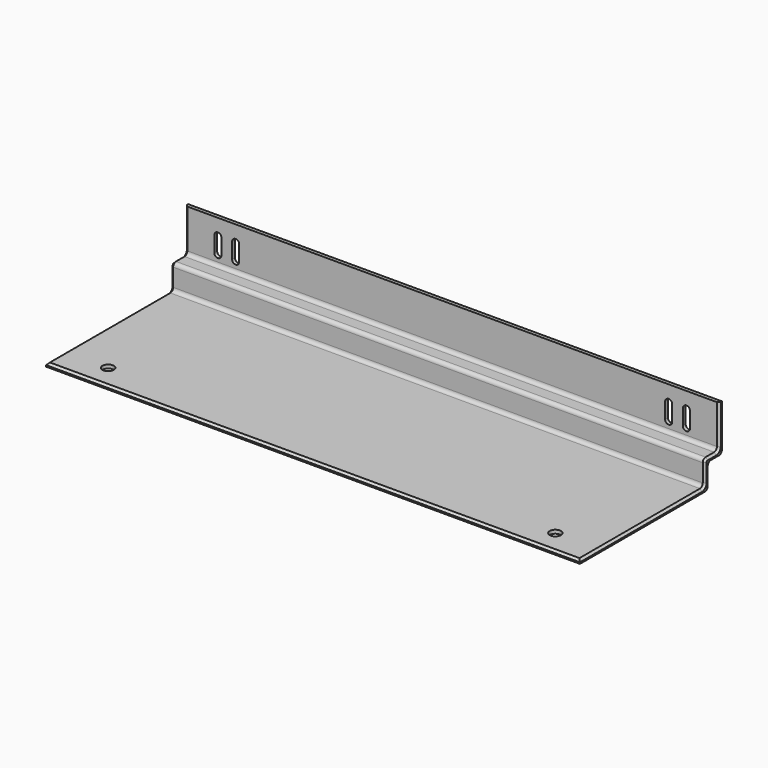
from build123d import *

# Parameters (mm, degrees)
F1_DEPTH     = 752
F3_DEPTH     = 5.001
F5_SIZE      = 3
F6_SIZE      = 3
F7_SIZE      = 3
F4_R         = 8
F8_DEPTH     = 25
F9_TEXT_SIZE = 16.7984515429
F10_DEPTH    = 0.5


# Not quite as in the source:
# - Text() gives the source's letters only with a copy of the font that has no kerning and outlines rounded to 1/6400 em; it was checked with that copy


with BuildPart() as f1:
    # F0 (on Right) → F1 (new body)
    with BuildSketch(Plane.YZ):
        with BuildLine():
            Line((0, -60), (0, 0))
            Line((0, 0), (-5, 0))
            Line((-5, 0), (-5, -55))
            ThreePointArc((-5, -55), (-6.4644660941, -58.5355339059), (-10, -60))
            Line((-10, -60), (-25, -60))
            ThreePointArc((-25, -60), (-28.5355339059, -61.4644660941), (-30, -65))
            Line((-30, -65), (-30, -90))
            ThreePointArc((-30, -90), (-31.4644660941, -93.5355339059), (-35, -95))
            Line((-35, -95), (-250, -95))
            Line((-250, -95), (-250, -100))
            Line((-250, -100), (-30, -100))
            ThreePointArc((-30, -100), (-26.4644660941, -98.5355339059), (-25, -95))
            Line((-25, -95), (-25, -70))
            ThreePointArc((-25, -70), (-23.5355339059, -66.4644660941), (-20, -65))
            Line((-20, -65), (-5, -65))
            ThreePointArc((-5, -65), (-1.4644660941, -63.5355339059), (0, -60))
        make_face()
    extrude(amount=F1_DEPTH)

    # F2 (on face) → F3 (cut, through all)
    with BuildSketch(Plane.XZ.offset(5)):
        with BuildLine():
            Line((686, -45), (686, -23))
            ThreePointArc((686, -23), (684.5355339059, -19.4644660941), (681, -18))
            ThreePointArc((681, -18), (677.4644660941, -19.4644660941), (676, -23))
            Line((676, -23), (676, -45))
            ThreePointArc((676, -45), (677.4644660941, -48.5355339059), (681, -50))
            ThreePointArc((681, -50), (684.5355339059, -48.5355339059), (686, -45))
        make_face()
        with BuildLine():
            Line((711, -45), (711, -23))
            ThreePointArc((711, -23), (709.5355339059, -19.4644660941), (706, -18))
            ThreePointArc((706, -18), (702.4644660941, -19.4644660941), (701, -23))
            Line((701, -23), (701, -45))
            ThreePointArc((701, -45), (702.4644660941, -48.5355339059), (706, -50))
            ThreePointArc((706, -50), (709.5355339059, -48.5355339059), (711, -45))
        make_face()
        with BuildLine():
            ThreePointArc((46, -50), (49.5355339059, -48.5355339059), (51, -45))
            Line((51, -45), (51, -23))
            ThreePointArc((51, -23), (49.5355339059, -19.4644660941), (46, -18))
            ThreePointArc((46, -18), (42.4644660941, -19.4644660941), (41, -23))
            Line((41, -23), (41, -45))
            ThreePointArc((41, -45), (42.4644660941, -48.5355339059), (46, -50))
        make_face()
        with BuildLine():
            ThreePointArc((66, -45), (67.4644660941, -48.5355339059), (71, -50))
            ThreePointArc((71, -50), (74.5355339059, -48.5355339059), (76, -45))
            Line((76, -45), (76, -23))
            ThreePointArc((76, -23), (74.5355339059, -19.4644660941), (71, -18))
            ThreePointArc((71, -18), (67.4644660941, -19.4644660941), (66, -23))
            Line((66, -23), (66, -45))
        make_face()
    extrude(amount=-F3_DEPTH, mode=Mode.SUBTRACT)

    # F5
    f5_edges = [f1.edges().sort_by_distance(p)[0] for p in [
        (376, -250, -95),
    ]]
    chamfer(f5_edges, length=F5_SIZE)

    # F6
    f6_edges = [f1.edges().sort_by_distance(p)[0] for p in [
        (0, -141, -95),
    ]]
    chamfer(f6_edges, length=F6_SIZE)

    # F7
    f7_edges = [f1.edges().sort_by_distance(p)[0] for p in [
        (752, -141, -95),
    ]]
    chamfer(f7_edges, length=F7_SIZE)

    # F4 (on face) → F8 (cut)
    with BuildSketch(Plane.XY.offset(-95)):
        with Locations((61, -217)):
            Circle(F4_R)
        with Locations((691, -217)):
            Circle(F4_R)
    extrude(amount=-F8_DEPTH, mode=Mode.SUBTRACT)

    # F9 (on face) → F10 (cut)
    with BuildSketch(Plane(origin=(0, 0, -100), x_dir=(1, 0, 0), z_dir=(0, 0, -1))):
        with Locations((594.0126776695, 36.5561470389)):
            Text('Regalboden 75 cm', F9_TEXT_SIZE, font='Open Sans', text_align=(TextAlign.LEFT, TextAlign.BOTTOM))
    extrude(amount=-F10_DEPTH, mode=Mode.SUBTRACT)


solid = f1.part
